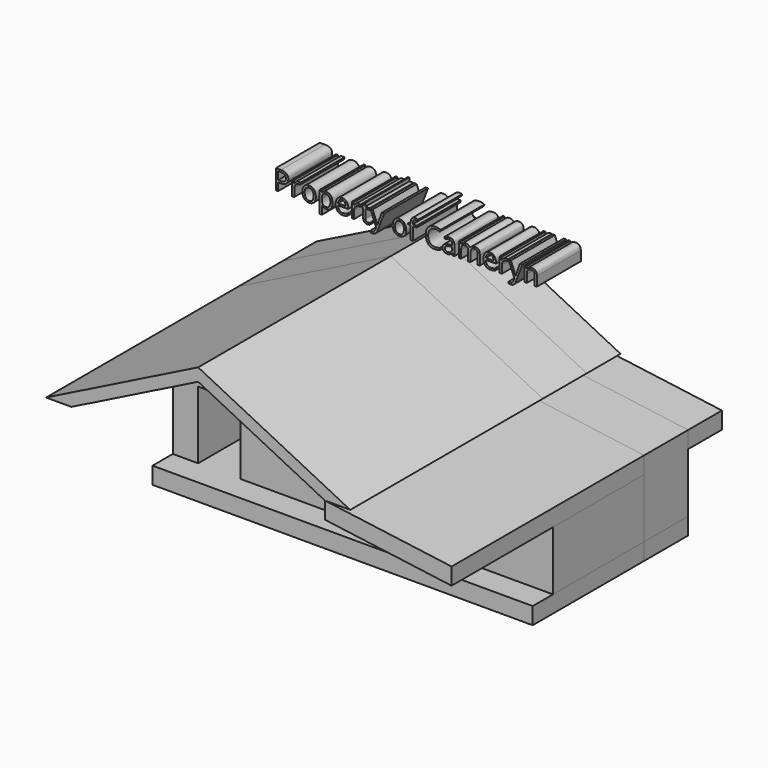
from build123d import *

# Parameters (mm, degrees)
F1_DEPTH      = 10668
F1_DEPTH_BACK = 1524
F2_DEPTH      = 1524
F2_DEPTH_BACK = 1524
F0_W          = 2743.2
F0_H          = 1371.6
F0_W_2        = 1219.2
F3_DEPTH      = 6096
F0_W_3        = 4572
F0_H_2        = 609.6
F4_DEPTH      = 7010.4
F0_W_4        = 2438.4
F0_H_3        = 1066.8
F0_W_5        = 914.4
F5_DEPTH      = 609.6
F0_TEXT_SIZE  = 986.7333703571
F6_DEPTH      = 1981.2


# Not quite as in the source:
# - Text() gives the source's letters only with a copy of the font that has no kerning and outlines rounded to 1/6400 em; it was checked with that copy


with BuildPart() as f1:
    # F0 (on Front) → F1 (new body, two sides)
    with BuildSketch(Plane.XZ) as f1_sk:
        Polygon((0, 2286), (4572, 0), (5486.4, 0), (0, 2743.2), align=None)
        Polygon((-5486.4, 0), (-4572, 0), (0, 2286), (0, 2743.2), align=None)
    extrude(amount=F1_DEPTH)
    extrude(f1_sk.sketch, amount=-F1_DEPTH_BACK)



with BuildPart() as f1b:
    # F0 (on Front) → F1, piece 2 (new body, two sides)
    with BuildSketch(Plane.XZ) as f1_2_sk:
        Polygon((9143.1556086981, -609.6001299571), (4572, 0), (4572, -609.6001299571), (9143.3432512096, -1219.2001010778), align=None)
    extrude(amount=F1_DEPTH)
    extrude(f1_2_sk.sketch, amount=-F1_DEPTH_BACK)


with BuildPart() as f1_1:
    add(f1.part)

    add(f1b.part)  # F2 merges F1b
    # F0 (on Front) → F2 (join, two sides)
    with BuildSketch(Plane.XZ) as f2_sk:
        Polygon((-4572, 0), (0, 0), (0, 2286), align=None)
        Polygon((0, 2286), (0, 0), (4572, 0), align=None)
    extrude(amount=F2_DEPTH)
    extrude(f2_sk.sketch, amount=-F2_DEPTH_BACK)


with BuildPart() as f3:
    # F0 (on Front) → F3 (new body)
    with BuildSketch(Plane.XZ):
        Polygon((4572, 0), (0, 0), (-4572, 0), (-4572, -3352.8), (-3657.6, -3352.8), (-3657.6, -914.4), (-2133.6, -914.4), (-2133.6, -3352.8), (4572, -3352.8), (4572, -609.6001299571), align=None)
        with Locations((1981.2, -1905)):
            Rectangle(F0_W, F0_H, mode=Mode.SUBTRACT)
        Polygon((9143.3432512096, -1219.2001010778), (4572, -609.6001299571), (4572, -3352.8), (9144, -3352.8), align=None)
        with Locations((6705.6, -1905)):
            Rectangle(F0_W_2, F0_H, mode=Mode.SUBTRACT)
    extrude(amount=F3_DEPTH)

    # F0 (on Front) → F4 (join)
    with BuildSketch(Plane.XZ):
        Polygon((-3657.6, -3352.8), (-4572, -3352.8), (-4572, -3962.4), (4572, -3962.4), (4572, -3352.8), (-2133.6, -3352.8), (-2438.4, -3352.8), (-3352.8, -3352.8), align=None)
        with Locations((6858, -3657.6)):
            Rectangle(F0_W_3, F0_H_2)
    extrude(amount=F4_DEPTH)

    # F0 (on Front) → F5 (join)
    with BuildSketch(Plane.XZ):
        Polygon((-3657.6, -914.4), (-3657.6, -3352.8), (-3352.8, -3352.8), (-3352.8, -1219.2), (-2438.4, -1219.2), (-2438.4, -3352.8), (-2133.6, -3352.8), (-2133.6, -914.4), align=None)
        with Locations((1981.2, -1905)):
            Rectangle(F0_W, F0_H)
        with Locations((1981.2, -1905)):
            Rectangle(F0_W_4, F0_H_3, mode=Mode.SUBTRACT)
        with Locations((6705.6, -1905)):
            Rectangle(F0_W_2, F0_H)
        with Locations((6705.6, -1905)):
            Rectangle(F0_W_5, F0_H_3, mode=Mode.SUBTRACT)
    extrude(amount=F5_DEPTH)


with BuildPart() as f6:
    # F0 (on Front) → F6 (new body)
    with BuildSketch(Plane.XZ):
        Polygon((4572, 0), (0, 0), (-4572, 0), (-4572, -3352.8), (-3657.6, -3352.8), (-3657.6, -914.4), (-2133.6, -914.4), (-2133.6, -3352.8), (4572, -3352.8), (4572, -609.6001299571), align=None)
        with Locations((1981.2, -1905)):
            Rectangle(F0_W, F0_H, mode=Mode.SUBTRACT)
        Polygon((0, 2286), (0, 0), (4572, 0), align=None)
        Polygon((-4572, 0), (0, 0), (0, 2286), align=None)
        Polygon((-5486.4, 0), (-4572, 0), (0, 2286), (0, 2743.2), align=None)
        Polygon((0, 2286), (4572, 0), (5486.4, 0), (0, 2743.2), align=None)
        Polygon((9143.1556086981, -609.6001299571), (4572, 0), (4572, -609.6001299571), (9143.3432512096, -1219.2001010778), align=None)
        Polygon((-3657.6, -3352.8), (-4572, -3352.8), (-4572, -3962.4), (4572, -3962.4), (4572, -3352.8), (-2133.6, -3352.8), (-2438.4, -3352.8), (-3352.8, -3352.8), align=None)
        Polygon((9143.3432512096, -1219.2001010778), (4572, -609.6001299571), (4572, -3352.8), (9144, -3352.8), align=None)
        with Locations((6705.6, -1905)):
            Rectangle(F0_W_2, F0_H, mode=Mode.SUBTRACT)
        with Locations((6858, -3657.6)):
            Rectangle(F0_W_3, F0_H_2)
        with Locations((-4240.7865524292, 3488.3382320404)):
            Text('Property of Cameryn', F0_TEXT_SIZE, font='Open Sans', text_align=(TextAlign.LEFT, TextAlign.BOTTOM))
    extrude(amount=F6_DEPTH)


solid = Compound([f1_1.part, f3.part, f6.part])
